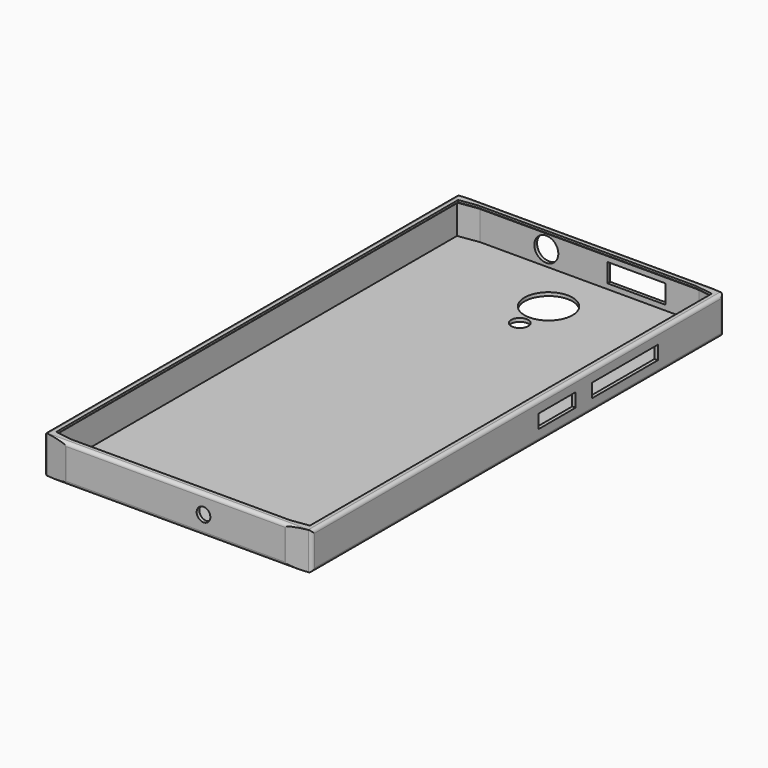
from build123d import *

# Parameters (mm, degrees)
F0_W        = 12
F0_H        = 4
F0_R        = 2.5
F0_R_2      = 7
F1_DEPTH    = 1
F3_DEPTH    = 8.9
F5_DEPTH    = 1
F6_T1_DEPTH = 155
F6_T3_DEPTH = 79
F6_T5_DEPTH = 11.2553390593
F6_T7_DEPTH = 15.2364770085
F7_SIZE     = 0.4
F8_W        = 13.5
F8_H        = 4
F8_W_2      = 24
F9_DEPTH    = 25
F10_R       = 3.5
F10_W       = 17
F10_H       = 5.5
F11_DEPTH   = 25
F12_R       = 2
F13_DEPTH   = 25


# Not quite as in the source:
# - a fillet or chamfer that OpenCascade refuses, or shapes differently, is made with other operations: its cross-section is extruded or revolved along the edge and cut away or added
# - a feature names something its author has since deleted; it is built from what else it names


with BuildPart() as f1:
    # F0 (on Top) → F1 (new body)
    with BuildSketch(Plane.XY):
        Polygon((32, 76), (-32, 76), (-39, 75), (-39, -75), (-32, -76), (32, -76), (39, -75), (39, 75), align=None)
        with Locations((0, -63)):
            Rectangle(F0_W, F0_H, mode=Mode.SUBTRACT)
        with Locations((0, 49.5)):
            Circle(F0_R, mode=Mode.SUBTRACT)
        with Locations((0, 60)):
            Circle(F0_R_2, mode=Mode.SUBTRACT)
    extrude(amount=F1_DEPTH)

    # F2 (on face) → F3 (join)
    with BuildSketch(Plane.XY.offset(1)):
        Polygon((39, 75), (32, 76), (-32, 76), (-39, 75), (-39, -75), (-32, -76), (32, -76), (39, -75), align=None)
        Polygon((31.9289321881, -75), (-31.9289321881, -75), (-38, -74.1327045983), (-38, 74.1327045983), (-31.9289321881, 75), (31.9289321881, 75), (38, 74.1327045983), (38, -74.1327045983), align=None, mode=Mode.SUBTRACT)
    extrude(amount=F3_DEPTH)

    # F4 (on face) → F5 (join)
    with BuildSketch(Plane.XY.offset(9.9)):
        Polygon((39, -75), (39, 75), (32, 76), (-32, 76), (-39, 75), (-39, -75), (-32, -76), (32, -76), align=None)
        Polygon((38, -74.1327045983), (31.9289321881, -75), (-31.9289321881, -75), (-38, -74.1327045983), (-38, 74.1327045983), (-31.9289321881, 75), (31.9289321881, 75), (38, 74.1327045983), align=None, mode=Mode.SUBTRACT)
        Polygon((-31.9289321881, -75), (31.9289321881, -75), (38, -74.1327045983), (38, 74.1327045983), (31.9289321881, 75), (-31.9289321881, 75), (-38, 74.1327045983), (-38, -74.1327045983), align=None)
        Polygon((-37, 73.2654091966), (-31.8578643763, 74), (31.8578643763, 74), (37, 73.2654091966), (37, -73.2654091966), (31.8578643763, -74), (-31.8578643763, -74), (-37, -73.2654091966), align=None, mode=Mode.SUBTRACT)
    extrude(amount=F5_DEPTH)

    # F6: fillet of radius 1 on 16 edges, made by hand

    # F6_s2 → F6_t1 (cut)
    with BuildSketch(Plane.XZ.offset(-77.5)):
        with BuildLine():
            ThreePointArc((-39, 9.9), (-38.7071067812, 10.6071067812), (-38, 10.9))
            Line((-38, 10.9), (-39, 10.9))
            Line((-39, 10.9), (-39, 9.9))
        make_face()
        with BuildLine():
            ThreePointArc((39, 9.9), (38.7071067812, 10.6071067812), (38, 10.9))
            Line((38, 10.9), (39, 10.9))
            Line((39, 10.9), (39, 9.9))
        make_face()
        with BuildLine():
            ThreePointArc((38, 0), (38.7071067812, 0.2928932188), (39, 1))
            Line((39, 1), (39, 0))
            Line((39, 0), (38, 0))
        make_face()
        with BuildLine():
            ThreePointArc((-38, 0), (-38.7071067812, 0.2928932188), (-39, 1))
            Line((-39, 1), (-39, 0))
            Line((-39, 0), (-38, 0))
        make_face()
    extrude(amount=F6_T1_DEPTH, mode=Mode.SUBTRACT)

    # F6_s4 → F6_t3 (cut)
    with BuildSketch(Plane.YZ.offset(-39.5)):
        with BuildLine():
            ThreePointArc((76, 9.9), (75.7071067812, 10.6071067812), (75, 10.9))
            Line((75, 10.9), (76, 10.9))
            Line((76, 10.9), (76, 9.9))
        make_face()
        with BuildLine():
            ThreePointArc((-76, 9.9), (-75.7071067812, 10.6071067812), (-75, 10.9))
            Line((-75, 10.9), (-76, 10.9))
            Line((-76, 10.9), (-76, 9.9))
        make_face()
        with BuildLine():
            ThreePointArc((-75, 0), (-75.7071067812, 0.2928932188), (-76, 1))
            Line((-76, 1), (-76, 0))
            Line((-76, 0), (-75, 0))
        make_face()
        with BuildLine():
            ThreePointArc((76, 1), (75.7071067812, 0.2928932188), (75, 0))
            Line((75, 0), (76, 0))
            Line((76, 0), (76, 1))
        make_face()
    extrude(amount=F6_T3_DEPTH, mode=Mode.SUBTRACT)

    # F6_s6 → F6_t5 (cut)
    with BuildSketch(Plane.XY.offset(-0.1776695297)):
        with BuildLine():
            ThreePointArc((31.9289321881, 76), (31.9998212082, 75.9974842088), (32.0703535444, 75.9899494937))
            Line((32.0703535444, 75.9899494937), (32, 76))
            Line((32, 76), (31.9289321881, 76))
        make_face()
        with BuildLine():
            ThreePointArc((-31.9289321881, 76), (-31.9998212082, 75.9974842088), (-32.0703535444, 75.9899494937))
            Line((-32.0703535444, 75.9899494937), (-32, 76))
            Line((-32, 76), (-31.9289321881, 76))
        make_face()
        with BuildLine():
            ThreePointArc((32.0703535444, -75.9899494937), (31.9998212082, -75.9974842088), (31.9289321881, -76))
            Line((31.9289321881, -76), (32, -76))
            Line((32, -76), (32.0703535444, -75.9899494937))
        make_face()
        with BuildLine():
            ThreePointArc((-31.9289321881, -76), (-31.9998212082, -75.9974842088), (-32.0703535444, -75.9899494937))
            Line((-32.0703535444, -75.9899494937), (-32, -76))
            Line((-32, -76), (-31.9289321881, -76))
        make_face()
    extrude(amount=F6_T5_DEPTH, mode=Mode.SUBTRACT)

    # F6_s8 → F6_t7 (cut)
    with BuildSketch(Plane.XY.offset(-2.1682385042)):
        with BuildLine():
            ThreePointArc((39, -74.1327045983), (38.755453955, -74.7879063397), (38.1414213562, -75.122654092))
            Line((38.1414213562, -75.122654092), (39, -75))
            Line((39, -75), (39, -74.1327045983))
        make_face()
        with BuildLine():
            ThreePointArc((39, 74.1327045983), (38.755453955, 74.7879063397), (38.1414213562, 75.122654092))
            Line((38.1414213562, 75.122654092), (39, 75))
            Line((39, 75), (39, 74.1327045983))
        make_face()
        with BuildLine():
            ThreePointArc((-38.1414213562, -75.122654092), (-38.755453955, -74.7879063397), (-39, -74.1327045983))
            Line((-39, -74.1327045983), (-39, -75))
            Line((-39, -75), (-38.1414213562, -75.122654092))
        make_face()
        with BuildLine():
            ThreePointArc((-39, 74.1327045983), (-38.755453955, 74.7879063397), (-38.1414213562, 75.122654092))
            Line((-38.1414213562, 75.122654092), (-39, 75))
            Line((-39, 75), (-39, 74.1327045983))
        make_face()
    extrude(amount=F6_T7_DEPTH, mode=Mode.SUBTRACT)

    # F7
    f7_edges = [f1.edges().sort_by_distance(p)[0] for p in [
        (-34.428932, 73.632705, 9.9),
        (-37, 0, 9.9),
        (0, 74, 9.9),
        (34.428932, 73.632705, 9.9),
        (37, 0, 9.9),
        (34.428932, -73.632705, 9.9),
        (0, -74, 9.9),
        (-34.428932, -73.632705, 9.9),
    ]]
    chamfer(f7_edges, length=F7_SIZE)

    # F8 (on face) → F9 (cut)
    with BuildSketch(Plane.YZ.offset(39)):
        with Locations((14.3827045983, 5.45)):
            Rectangle(F8_W, F8_H)
        with Locations((39.1327045983, 5.45)):
            Rectangle(F8_W_2, F8_H)
    extrude(amount=-F9_DEPTH, mode=Mode.SUBTRACT)

    # F10 (on face) → F11 (cut)
    with BuildSketch(Plane(origin=(0, 76, 0), x_dir=(-1, 0, 0), z_dir=(0, 1, 0))):
        with Locations((12.6414213562, 5.45)):
            Circle(F10_R)
        with Locations((-13.6414213562, 5.25)):
            Rectangle(F10_W, F10_H)
    extrude(amount=-F11_DEPTH, mode=Mode.SUBTRACT)

    # F12 (on face) → F13 (cut)
    with BuildSketch(Plane.XZ.offset(76)):
        with Locations((8.1414213562, 5.45)):
            Circle(F12_R)
    extrude(amount=-F13_DEPTH, mode=Mode.SUBTRACT)


solid = f1.part
